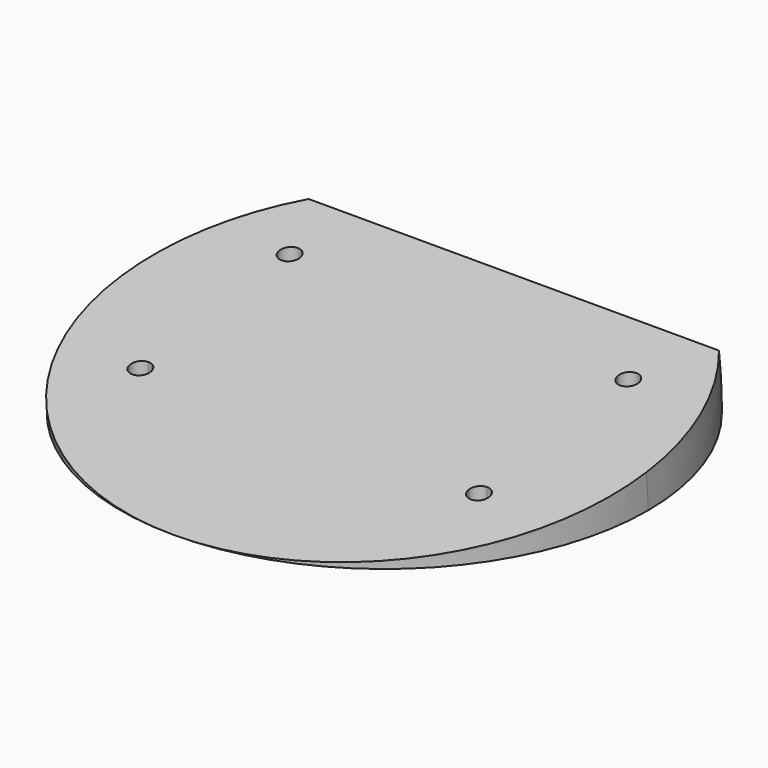
from build123d import *

# Parameters (mm, degrees)
F1_ANGLE = 7.5
F2_DEPTH = 13.8130175157


# Not quite as in the source:
# - a feature names something its author has since deleted; it is built from what else it names


with BuildPart() as f1:
    # F0 (on Top) → F1 (revolve)
    with BuildSketch(Plane.XY):
        with BuildLine():
            ThreePointArc((0, -65), (45.9619407771, -45.9619407771), (65, 0))
            ThreePointArc((65, 0), (61.2905274084, 21.6441966818), (50.5855, 40.8179763064))
            Line((50.5855, 40.8179763064), (-50.5855, 40.8179763064))
            ThreePointArc((-50.5855, 40.8179763064), (-58.6437058, -28.034189306), (0, -65))
        make_face()
        with BuildLine():
            Line((39.25, -23), (-39.25, -23))
            ThreePointArc((-39.25, -23), (-43.517766953, -24.767766953), (-41.75, -20.5))
            Line((-41.75, -20.5), (-41.75, 20.5))
            ThreePointArc((-41.75, 20.5), (-43.517766953, 24.767766953), (-39.25, 23))
            Line((-39.25, 23), (39.25, 23))
            ThreePointArc((39.25, 23), (41.75, 25.5), (44.25, 23))
            ThreePointArc((44.25, 23), (43.517766953, 21.232233047), (41.75, 20.5))
            Line((41.75, 20.5), (41.75, -20.5))
            ThreePointArc((41.75, -20.5), (43.517766953, -21.232233047), (44.25, -23))
            ThreePointArc((44.25, -23), (41.75, -25.5), (39.25, -23))
        make_face(mode=Mode.SUBTRACT)
        with BuildLine():
            ThreePointArc((-41.75, -20.5), (-43.517766953, -24.767766953), (-39.25, -23))
            Line((-39.25, -23), (-41.75, -23))
            Line((-41.75, -23), (-41.75, -20.5))
        make_face()
        with BuildLine():
            ThreePointArc((-41.75, -20.5), (-39.982233047, -21.232233047), (-39.25, -23))
            Line((-39.25, -23), (39.25, -23))
            ThreePointArc((39.25, -23), (39.982233047, -21.232233047), (41.75, -20.5))
            Line((41.75, -20.5), (41.75, 20.5))
            ThreePointArc((41.75, 20.5), (39.982233047, 21.232233047), (39.25, 23))
            Line((39.25, 23), (-39.25, 23))
            ThreePointArc((-39.25, 23), (-39.982233047, 21.232233047), (-41.75, 20.5))
            Line((-41.75, 20.5), (-41.75, -20.5))
        make_face()
        with BuildLine():
            Line((-41.75, -23), (-39.25, -23))
            ThreePointArc((-39.25, -23), (-39.982233047, -21.232233047), (-41.75, -20.5))
            Line((-41.75, -20.5), (-41.75, -23))
        make_face()
        with BuildLine():
            ThreePointArc((41.75, -20.5), (39.982233047, -21.232233047), (39.25, -23))
            Line((39.25, -23), (41.75, -23))
            Line((41.75, -23), (41.75, -20.5))
        make_face()
        with BuildLine():
            Line((41.75, -23), (39.25, -23))
            ThreePointArc((39.25, -23), (41.75, -25.5), (44.25, -23))
            ThreePointArc((44.25, -23), (43.517766953, -21.232233047), (41.75, -20.5))
            Line((41.75, -20.5), (41.75, -23))
        make_face()
        with BuildLine():
            ThreePointArc((-39.25, 23), (-43.517766953, 24.767766953), (-41.75, 20.5))
            Line((-41.75, 20.5), (-41.75, 23))
            Line((-41.75, 23), (-39.25, 23))
        make_face()
        with BuildLine():
            Line((-41.75, 23), (-41.75, 20.5))
            ThreePointArc((-41.75, 20.5), (-39.982233047, 21.232233047), (-39.25, 23))
            Line((-39.25, 23), (-41.75, 23))
        make_face()
        with BuildLine():
            ThreePointArc((39.25, 23), (39.982233047, 21.232233047), (41.75, 20.5))
            Line((41.75, 20.5), (41.75, 23))
            Line((41.75, 23), (39.25, 23))
        make_face()
        with BuildLine():
            Line((41.75, 23), (41.75, 20.5))
            ThreePointArc((41.75, 20.5), (43.517766953, 21.232233047), (44.25, 23))
            ThreePointArc((44.25, 23), (41.75, 25.5), (39.25, 23))
            Line((39.25, 23), (41.75, 23))
        make_face()
    revolve(axis=Axis((33.3227813244, -65, 0), (1, 0, 0)), revolution_arc=F1_ANGLE)

    # F0 (on Top) → F2 (cut, through all)
    with BuildSketch(Plane.XY):
        with BuildLine():
            Line((-41.75, -23), (-39.25, -23))
            ThreePointArc((-39.25, -23), (-39.982233047, -21.232233047), (-41.75, -20.5))
            Line((-41.75, -20.5), (-41.75, -23))
        make_face()
        with BuildLine():
            ThreePointArc((-41.75, -20.5), (-43.517766953, -24.767766953), (-39.25, -23))
            Line((-39.25, -23), (-41.75, -23))
            Line((-41.75, -23), (-41.75, -20.5))
        make_face()
        with BuildLine():
            ThreePointArc((41.75, -20.5), (39.982233047, -21.232233047), (39.25, -23))
            Line((39.25, -23), (41.75, -23))
            Line((41.75, -23), (41.75, -20.5))
        make_face()
        with BuildLine():
            Line((41.75, -23), (39.25, -23))
            ThreePointArc((39.25, -23), (41.75, -25.5), (44.25, -23))
            ThreePointArc((44.25, -23), (43.517766953, -21.232233047), (41.75, -20.5))
            Line((41.75, -20.5), (41.75, -23))
        make_face()
        with BuildLine():
            ThreePointArc((39.25, 23), (39.982233047, 21.232233047), (41.75, 20.5))
            Line((41.75, 20.5), (41.75, 23))
            Line((41.75, 23), (39.25, 23))
        make_face()
        with BuildLine():
            Line((41.75, 23), (41.75, 20.5))
            ThreePointArc((41.75, 20.5), (43.517766953, 21.232233047), (44.25, 23))
            ThreePointArc((44.25, 23), (41.75, 25.5), (39.25, 23))
            Line((39.25, 23), (41.75, 23))
        make_face()
        with BuildLine():
            Line((-41.75, 23), (-41.75, 20.5))
            ThreePointArc((-41.75, 20.5), (-39.982233047, 21.232233047), (-39.25, 23))
            Line((-39.25, 23), (-41.75, 23))
        make_face()
        with BuildLine():
            ThreePointArc((-39.25, 23), (-43.517766953, 24.767766953), (-41.75, 20.5))
            Line((-41.75, 20.5), (-41.75, 23))
            Line((-41.75, 23), (-39.25, 23))
        make_face()
    extrude(amount=F2_DEPTH, mode=Mode.SUBTRACT)


solid = f1.part
